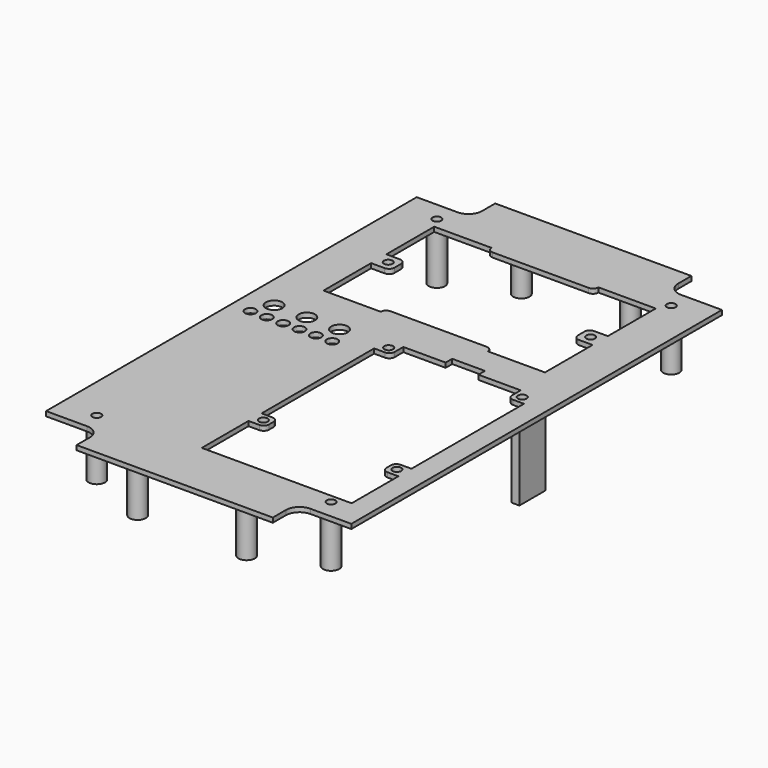
from build123d import *

# Parameters (mm, degrees)
F0_R     = 1.6
F0_R_2   = 2
F0_R_3   = 3
F2_DEPTH = 1.7
F3_R     = 1.6
F4_DEPTH = 1.701
F5_R     = 3
F5_R_2   = 1.6
F6_DEPTH = 19
F1_R     = 1.5875
F7_DEPTH = 20.701
F5_W     = 3
F5_H     = 12
F8_DEPTH = 25


# Not quite as in the source:
# - a feature names something its author has since deleted; it is built from what else it names


with BuildPart() as f2:
    # F0 (on Top) → F2 (new body)
    with BuildSketch(Plane.XY):
        with BuildLine():
            Line((36, 90), (36, 96))
            Line((36, 96), (-36, 96))
            Line((-36, 96), (-36, 90))
            ThreePointArc((-36, 90), (-37.4644660941, 86.4644660941), (-41, 85))
            Line((-41, 85), (-56, 85))
            Line((-56, 85), (-56, -85))
            Line((-56, -85), (-41, -85))
            ThreePointArc((-41, -85), (-37.4644660941, -86.4644660941), (-36, -90))
            Line((-36, -90), (-36, -96))
            Line((-36, -96), (36, -96))
            Line((36, -96), (36, -90))
            ThreePointArc((36, -90), (37.4644660941, -86.4644660941), (41, -85))
            Line((41, -85), (56, -85))
            Line((56, -85), (56, 85))
            Line((56, 85), (41, 85))
            ThreePointArc((41, 85), (37.4644660941, 86.4644660941), (36, 90))
        make_face()
        with Locations((-43, -78)):
            Circle(F0_R, mode=Mode.SUBTRACT)
        with Locations((43, -78)):
            Circle(F0_R, mode=Mode.SUBTRACT)
        with Locations((-49, 0)):
            Circle(F0_R_2, mode=Mode.SUBTRACT)
        with Locations((-43, 0)):
            Circle(F0_R_2, mode=Mode.SUBTRACT)
        with Locations((-46, 7.1000065655)):
            Circle(F0_R_3, mode=Mode.SUBTRACT)
        with Locations((-37, 0)):
            Circle(F0_R_2, mode=Mode.SUBTRACT)
        with Locations((-31, 0)):
            Circle(F0_R_2, mode=Mode.SUBTRACT)
        with Locations((-34, 7.0999998483)):
            Circle(F0_R_3, mode=Mode.SUBTRACT)
        with Locations((-25, 0)):
            Circle(F0_R_2, mode=Mode.SUBTRACT)
        with Locations((-22, 7.0999931312)):
            Circle(F0_R_3, mode=Mode.SUBTRACT)
        with Locations((-19, 0)):
            Circle(F0_R_2, mode=Mode.SUBTRACT)
        with Locations((-43, 78)):
            Circle(F0_R, mode=Mode.SUBTRACT)
        with Locations((43, 78)):
            Circle(F0_R, mode=Mode.SUBTRACT)
    extrude(amount=-F2_DEPTH)

    # F3 (on face) → F4 (cut, through all)
    with BuildSketch(Plane.XY):
        with BuildLine():
            Line((-6.8923553079, -74.973076582), (48.1076446921, -74.973076582))
            Line((48.1076446921, -74.973076582), (48.1076446921, -53.5361680277))
            Line((48.1076446921, -53.5361680277), (44.1514502317, -53.5361680277))
            ThreePointArc((44.1514502317, -53.5361680277), (42.7372366693, -52.95038159), (42.1514502317, -51.5361680277))
            Line((42.1514502317, -51.5361680277), (42.1514502317, -49.5361680277))
            ThreePointArc((42.1514502317, -49.5361680277), (42.7372366693, -48.1219544653), (44.1514502317, -47.5361680277))
            Line((44.1514502317, -47.5361680277), (48.1076446921, -47.5361680277))
            Line((48.1076446921, -47.5361680277), (48.1076446921, 4.0900148638))
            Line((48.1076446921, 4.0900148638), (44.1514502317, 4.0900148638))
            ThreePointArc((44.1514502317, 4.0900148638), (42.7372366693, 4.6758013014), (42.1514502317, 6.0900148638))
            Line((42.1514502317, 6.0900148638), (42.1514502317, 10.026923418))
            Line((42.1514502317, 10.026923418), (26.6076446921, 10.026923418))
            Line((26.6076446921, 10.026923418), (26.6076446921, 13.026923418))
            Line((26.6076446921, 13.026923418), (14.6076446921, 13.026923418))
            Line((14.6076446921, 13.026923418), (14.6076446921, 10.026923418))
            Line((14.6076446921, 10.026923418), (-0.9361608475, 10.026923418))
            Line((-0.9361608475, 10.026923418), (-0.9361608475, 6.0900148638))
            ThreePointArc((-0.9361608475, 6.0900148638), (-1.5219472852, 4.6758013014), (-2.9361608475, 4.0900148638))
            Line((-2.9361608475, 4.0900148638), (-6.8923553079, 4.0900148638))
            Line((-6.8923553079, 4.0900148638), (-6.8923553079, -47.5361680277))
            Line((-6.8923553079, -47.5361680277), (-2.9361608475, -47.5361680277))
            ThreePointArc((-2.9361608475, -47.5361680277), (-1.5219472852, -48.1219544653), (-0.9361608475, -49.5361680277))
            Line((-0.9361608475, -49.5361680277), (-0.9361608475, -51.5361680277))
            ThreePointArc((-0.9361608475, -51.5361680277), (-1.5219472852, -52.95038159), (-2.9361608475, -53.5361680277))
            Line((-2.9361608475, -53.5361680277), (-6.8923553079, -53.5361680277))
            Line((-6.8923553079, -53.5361680277), (-6.8923553079, -74.973076582))
        make_face()
        with Locations((-3.8923553079, -50.473076582)):
            Circle(F3_R)
        with Locations((45.1076446921, -50.473076582)):
            Circle(F3_R)
        with Locations((-3.8923553079, 7.026923418)):
            Circle(F3_R)
        with Locations((45.1076446921, 7.026923418)):
            Circle(F3_R)
    extrude(amount=-F4_DEPTH, mode=Mode.SUBTRACT)

    # F5 (on face) → F6 (join)
    with BuildSketch(Plane(origin=(0, 0, -1.7), x_dir=(1, 0, 0), z_dir=(0, 0, -1))):
        with Locations((-20, 88)):
            Circle(F5_R)
        with Locations((20, 88)):
            Circle(F5_R)
        with Locations((-20, -88)):
            Circle(F5_R)
        with Locations((20, -88)):
            Circle(F5_R)
        with Locations((-43, 78)):
            Circle(F5_R)
        with Locations((-43, 78)):
            Circle(F5_R_2, mode=Mode.SUBTRACT)
        with Locations((43, 78)):
            Circle(F5_R)
        with Locations((43, 78)):
            Circle(F5_R_2, mode=Mode.SUBTRACT)
        with Locations((43, -78)):
            Circle(F5_R)
        with Locations((43, -78)):
            Circle(F5_R_2, mode=Mode.SUBTRACT)
        with Locations((-43, -78)):
            Circle(F5_R)
        with Locations((-43, -78)):
            Circle(F5_R_2, mode=Mode.SUBTRACT)
    extrude(amount=F6_DEPTH)

    # F1 (on face) → F7 (cut, through all)
    with BuildSketch(Plane.XY):
        with BuildLine():
            Line((-40.6379473025, 44.8732740056), (-40.6379473025, 23.0366364121))
            Line((-40.6379473025, 23.0366364121), (-19.6368917197, 23.0366364121))
            ThreePointArc((-19.6368917197, 23.0366364121), (-19.0511052821, 24.4508499745), (-17.6368917197, 25.0366364121))
            Line((-17.6368917197, 25.0366364121), (17.6409971148, 25.0366364121))
            ThreePointArc((17.6409971148, 25.0366364121), (19.0552106772, 24.4508499745), (19.6409971148, 23.0366364121))
            Line((19.6409971148, 23.0366364121), (40.6420526975, 23.0366364121))
            Line((40.6420526975, 23.0366364121), (40.6420526975, 44.8732740056))
            Line((40.6420526975, 44.8732740056), (35.6420526975, 44.8732740056))
            ThreePointArc((35.6420526975, 44.8732740056), (34.2278391352, 45.4590604432), (33.6420526975, 46.8732740056))
            Line((33.6420526975, 46.8732740056), (33.6420526975, 49.8732740056))
            ThreePointArc((33.6420526975, 49.8732740056), (34.2278391352, 51.287487568), (35.6420526975, 51.8732740056))
            Line((35.6420526975, 51.8732740056), (40.6420526975, 51.8732740056))
            Line((40.6420526975, 51.8732740056), (40.6420526975, 73.8366364121))
            Line((40.6420526975, 73.8366364121), (19.6409971148, 73.8366364121))
            ThreePointArc((19.6409971148, 73.8366364121), (19.0552106772, 72.4224228498), (17.6409971148, 71.8366364121))
            Line((17.6409971148, 71.8366364121), (-17.6368917197, 71.8366364121))
            ThreePointArc((-17.6368917197, 71.8366364121), (-19.0511052821, 72.4224228498), (-19.6368917197, 73.8366364121))
            Line((-19.6368917197, 73.8366364121), (-40.6379473025, 73.8366364121))
            Line((-40.6379473025, 73.8366364121), (-40.6379473025, 51.8732740056))
            Line((-40.6379473025, 51.8732740056), (-35.6379473025, 51.8732740056))
            ThreePointArc((-35.6379473025, 51.8732740056), (-34.2237337401, 51.287487568), (-33.6379473025, 49.8732740056))
            Line((-33.6379473025, 49.8732740056), (-33.6379473025, 46.8732740056))
            ThreePointArc((-33.6379473025, 46.8732740056), (-34.2237337401, 45.4590604432), (-35.6379473025, 44.8732740056))
            Line((-35.6379473025, 44.8732740056), (-40.6379473025, 44.8732740056))
        make_face()
        with Locations((-37.1379473025, 48.3732740056)):
            Circle(F1_R)
        with Locations((37.1379473025, 48.3732740056)):
            Circle(F1_R)
    extrude(amount=-F7_DEPTH, mode=Mode.SUBTRACT)

    # F5 (on face) → F8 (join)
    with BuildSketch(Plane(origin=(0, 0, -1.7), x_dir=(1, 0, 0), z_dir=(0, 0, -1))):
        with Locations((53, 0)):
            Rectangle(F5_W, F5_H)
        with Locations((-53, 0)):
            Rectangle(F5_W, F5_H)
    extrude(amount=F8_DEPTH)


solid = f2.part
